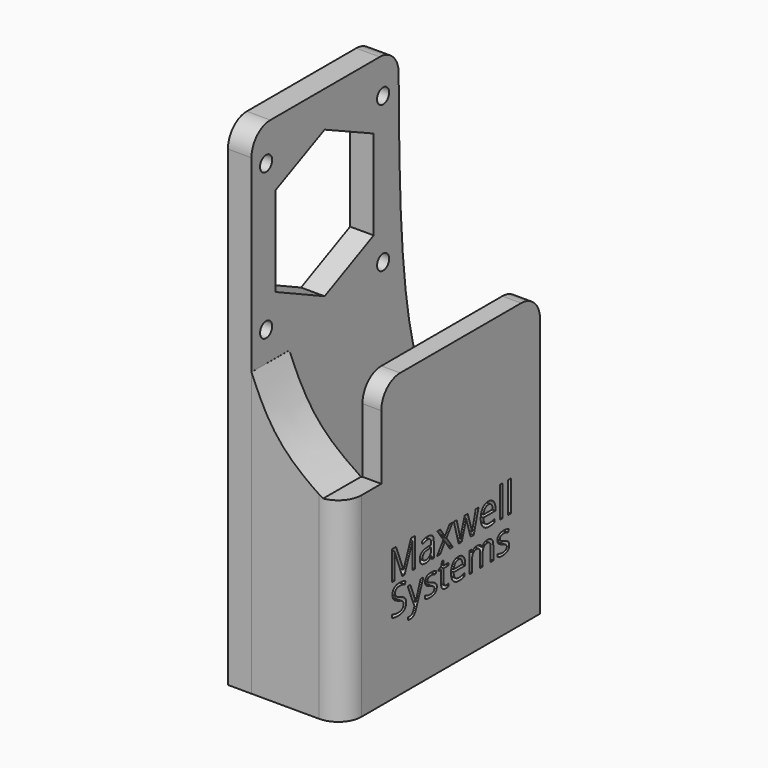
from build123d import *

# Parameters (mm, degrees)
F1_DEPTH        = 105
F2_R            = 1.5
F3_DEPTH        = 26
F4_R            = 1.6
F5_DEPTH        = 25
F6_R            = 5
F7_DEPTH        = 60
F9_DEPTH        = 10.2
F10_F1_R        = 5
F10_F2_R        = 5
F10_F3_R        = 5
F11_TEXT_SIZE   = 8.6434495946
F11_TEXT_SIZE_2 = 8.2639770375
F12_DEPTH       = 4


# Not quite as in the source:
# - a feature names something its author has since deleted; it is built from what else it names
# - Text() gives the source's letters only with a copy of the font that has no kerning and outlines rounded to 1/6400 em; it was checked with that copy


with BuildPart() as f1:
    # F0 (on Top) → F1 (new body)
    with BuildSketch(Plane.XY):
        Polygon((-20.2, -10.2), (-15.2, -10.2167241275), (-15.2, -0.2), (-15.2, -0.0167241275), (-15.2, 0), (-15.2, 42), (-20.2, 42), (-20.2, 0), align=None)
    extrude(amount=F1_DEPTH)

    # F2 (on face) → F3 (cut)
    with BuildSketch(Plane(origin=(-20.2, 0, 0), x_dir=(0, -1, 0), z_dir=(-1, 0, 0))):
        with Locations((-36.5, 7.75)):
            Circle(F2_R)
        with Locations((-5.5, 7.75)):
            Circle(F2_R)
    extrude(amount=-F3_DEPTH, mode=Mode.SUBTRACT)

    # F4 (on face) → F5 (cut)
    with BuildSketch(Plane(origin=(-20.2, 0, 0), x_dir=(0, -1, 0), z_dir=(-1, 0, 0))):
        with BuildLine():
            Line((-42, 105), (-42, 23.1413375586))
            add(Edge.make_bspline(
                [(-42, 23.1413375586), (-38.276727379, 31.6940768224), (-28.2913886113, 51.0818409085), (-28.9516502963, 90.9725008059), (-28.7173148245, 105)],
                knots=[0, 0, 0, 0, 0.4343083423, 1, 1, 1, 1], degree=3))
            Line((-28.7173148245, 105), (-42, 105))
        make_face()
        with Locations((-24.6643323809, 97.3597530909)):
            Circle(F4_R)
        with Locations((6.3356676191, 97.3597530909)):
            Circle(F4_R)
        with Locations((6.3356676191, 66.3597530909)):
            Circle(F4_R)
        with Locations((-24.6643323809, 66.3597530909)):
            Circle(F4_R)
        Polygon((-22.1648292974, 91.3592589684), (-22.1648292974, 74.8680422492), (-22.1648292974, 72.3592589684), (-9.1648292974, 66.2850100137), (3.8351707026, 72.3592589684), (3.8351707026, 74.8680422492), (3.8351707026, 91.3592589684), (-9.1648292974, 97.3677910455), align=None)
    extrude(amount=-F5_DEPTH, mode=Mode.SUBTRACT)

    # F6
    f6_edges = [f1.edges().sort_by_distance(p)[0] for p in [
        (-17.7, 28.717315, 105),
        (-17.7, -10.208362, 105),
        (-17.7, 42, 23.141338),
    ]]
    fillet(f6_edges, radius=F6_R)

    # F0 (on Top) → F7 (join)
    with BuildSketch(Plane.XY):
        Polygon((4.2, 42), (0.2, 42), (0.2, 41.8880863234), (0.2, 0), (0.2, -0.2), (0, -0.2), (-15, -0.2), (-15.2, -0.2), (-15.2, -10.2167241275), (4.2, -10.2675654752), (4.2, 41.8880863234), align=None)
    extrude(amount=F7_DEPTH)

    # F8 (on face) → F9 (cut)
    with BuildSketch(Plane(origin=(-0.0268790557, -10.2564881439, 0), x_dir=(0.999996566, -0.002620679, 0), z_dir=(-0.002620679, -0.999996566, 0))):
        with BuildLine():
            Line((0, 60), (-15.1731730488, 60))
            add(Edge.make_bspline(
                [(-15.1731730488, 60), (-13.1862126131, 55.3061912792), (-10.3567252223, 48.6220760085), (-2.0707267797, 42.6885437094), (0, 41.3452484289)],
                knots=[0, 0, 0, 0, 0.4955467448, 0.7056724638, 0.7056724638, 0.7056724638, 0.7056724638], degree=3))
            Line((0, 41.3452484289), (4.2268935708, 41.3452484289))
            Line((4.2268935708, 41.3452484289), (4.2268935708, 60))
            Line((4.2268935708, 60), (0, 60))
        make_face()
        with BuildLine():
            add(Edge.make_bspline(
                [(4.2268935708, 38.9642119408), (4.2214544117, 38.9904774991), (4.2241739912, 39.020681022), (4.2268935708, 39.0508845448)],
                knots=[0.9637675025, 0.9637675025, 0.9637675025, 0.9637675025, 1, 1, 1, 1], degree=3))
            Line((4.2268935708, 38.9642119408), (4.2268935708, 39.0508845448))
        make_face()
    extrude(amount=-F9_DEPTH, mode=Mode.SUBTRACT)

    # F10: fillet of radius 5 on 4 edges, made by hand

    # F10_f1
    f10_f1_edges = [f1.edges().sort_by_distance(p)[0] for p in [
        (4.2, -10.2675654752, 40.1980664869),
    ]]
    fillet(f10_f1_edges, radius=F10_F1_R)

    # F10_f2
    f10_f2_edges = [f1.edges().sort_by_distance(p)[0] for p in [
        (2.2, 42, 60),
    ]]
    fillet(f10_f2_edges, radius=F10_F2_R)

    # F10_f3
    f10_f3_edges = [f1.edges().sort_by_distance(p)[0] for p in [
        (2.2, -0.0622890724, 60),
    ]]
    fillet(f10_f3_edges, radius=F10_F3_R)

    # F11 (on face) → F12 (cut)
    with BuildSketch(Plane.YZ.offset(4.2)):
        with Locations((1.9231400043, 21.8358318472)):
            Text('Maxwell', F11_TEXT_SIZE, font='Open Sans', text_align=(TextAlign.LEFT, TextAlign.BOTTOM))
        with Locations((2.3836100043, 14.9594183802)):
            Text('Systems', F11_TEXT_SIZE_2, font='Open Sans', text_align=(TextAlign.LEFT, TextAlign.BOTTOM))
    extrude(amount=-F12_DEPTH, mode=Mode.SUBTRACT)


solid = f1.part
